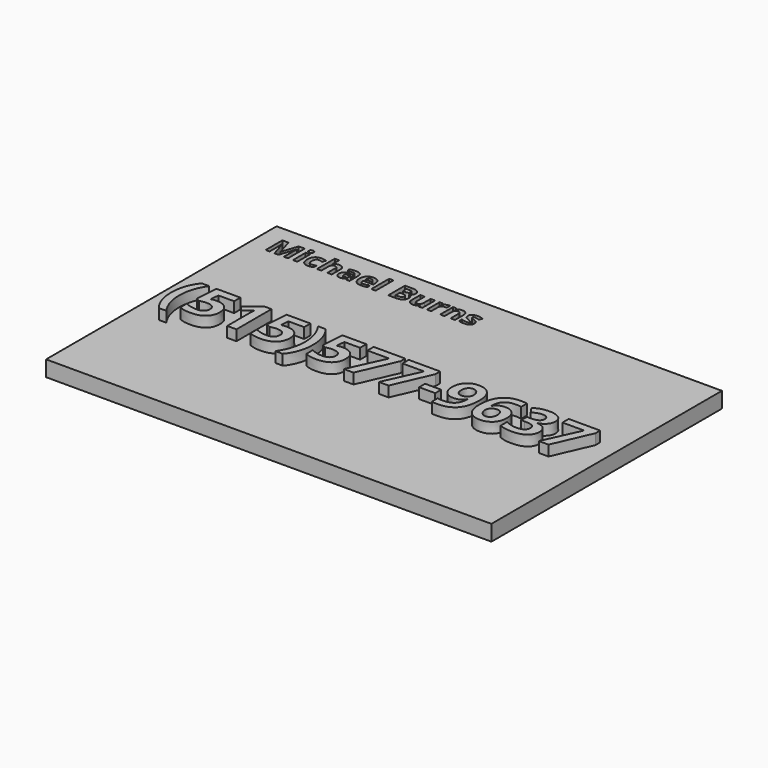
from build123d import *

# Parameters (mm, degrees)
F0_W         = 85
F0_H         = 55
F1_DEPTH     = 3
F2_TEXT_SIZE = 5.599545037
F3_DEPTH     = 2
F4_TEXT_SIZE = 11.7202531352
F5_DEPTH     = 2


# Not quite as in the source:
# - Text() gives the source's letters only with a copy of the font that has no kerning and outlines rounded to 1/6400 em; it was checked with that copy


with BuildPart() as f1:
    # F0 (on Top) → F1 (new body)
    with BuildSketch(Plane.XY):
        Rectangle(F0_W, F0_H)
    extrude(amount=F1_DEPTH)

    # F2 (on face) → F3 (cut)
    with BuildSketch(Plane.XY.offset(3)):
        with Locations((-39.5, 20.5)):
            Text('Michael Burns', F2_TEXT_SIZE, font='Open Sans', font_style=FontStyle.BOLD, text_align=(TextAlign.LEFT, TextAlign.BOTTOM))
    extrude(amount=-F3_DEPTH, mode=Mode.SUBTRACT)

    # F4 (on face) → F5 (join)
    with BuildSketch(Plane.XY.offset(3)):
        with Locations((-39.5, -5.2149957573)):
            Text('(515)577-9637', F4_TEXT_SIZE, font='Open Sans', font_style=FontStyle.BOLD, text_align=(TextAlign.LEFT, TextAlign.BOTTOM))
    extrude(amount=F5_DEPTH)


solid = f1.part
